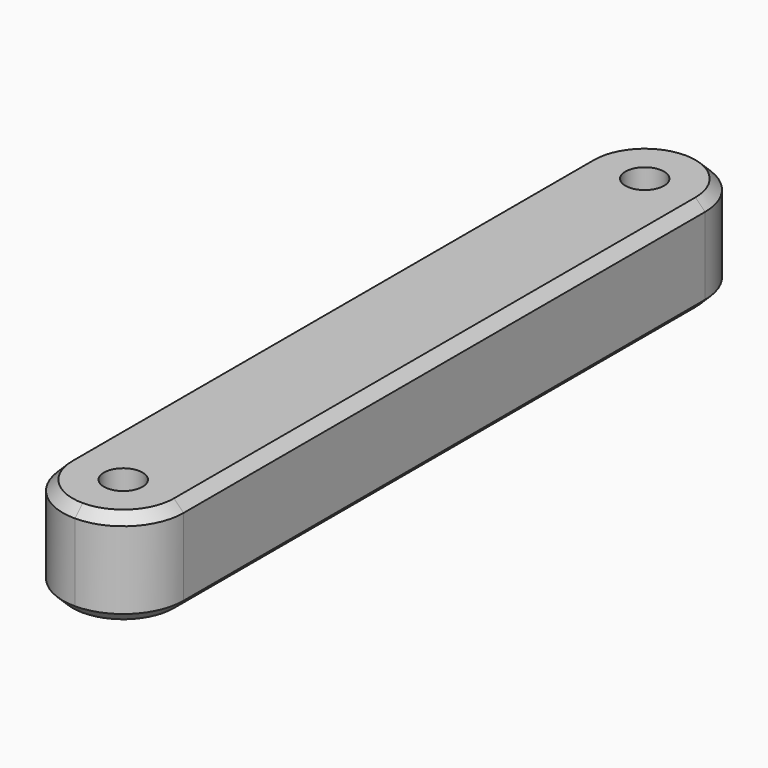
from build123d import *

# Parameters (mm, degrees)
F0_W     = 12.5
F0_H     = 10
F1_DEPTH = 80
F2_R     = 2
F3_DEPTH = 10
F4_R     = 6.24999
F5_SIZE  = 1


# Not quite as in the source:
# - a fillet or chamfer is up to 0.001 mm smaller than in the source, because OpenCascade refuses the exact size


with BuildPart() as f1:
    # F0 (on Front) → F1 (new body)
    with BuildSketch(Plane.XZ):
        with Locations((6.25, 5)):
            Rectangle(F0_W, F0_H)
    extrude(amount=-F1_DEPTH)

    # F2 (on face) → F3 (cut, through all)
    with BuildSketch(Plane.XY.offset(10)):
        with Locations((6.25, 73.75)):
            Circle(F2_R)
        with Locations((6.25, 6.25)):
            Circle(F2_R)
    extrude(amount=-F3_DEPTH, mode=Mode.SUBTRACT)

    # F4 (radius 6.25 in the source; OpenCascade refuses exactly that, so slightly less here)
    f4_edges = [f1.edges().sort_by_distance(p)[0] for p in [
        (12.5, 0, 5),
        (0, 0, 5),
        (12.5, 80, 5),
        (0, 80, 5),
    ]]
    fillet(f4_edges, radius=F4_R)

    # F5
    f5_edges = [f1.edges().sort_by_distance(p)[0] for p in [
        (0, 40, 10),
        (0, 6.24999, 5),
        (0, 73.75001, 5),
        (0, 40, 0),
        (10.66942, 1.83058, 0),
        (6.25001, 0, 5),
        (12.5, 6.24999, 5),
        (10.66942, 1.83058, 10),
        (12.5, 40, 0),
        (12.5, 73.75001, 5),
        (12.5, 40, 10),
        (10.66942, 78.16942, 0),
        (6.25001, 80, 5),
        (10.66942, 78.16942, 10),
    ]]
    chamfer(f5_edges, length=F5_SIZE)


solid = f1.part
